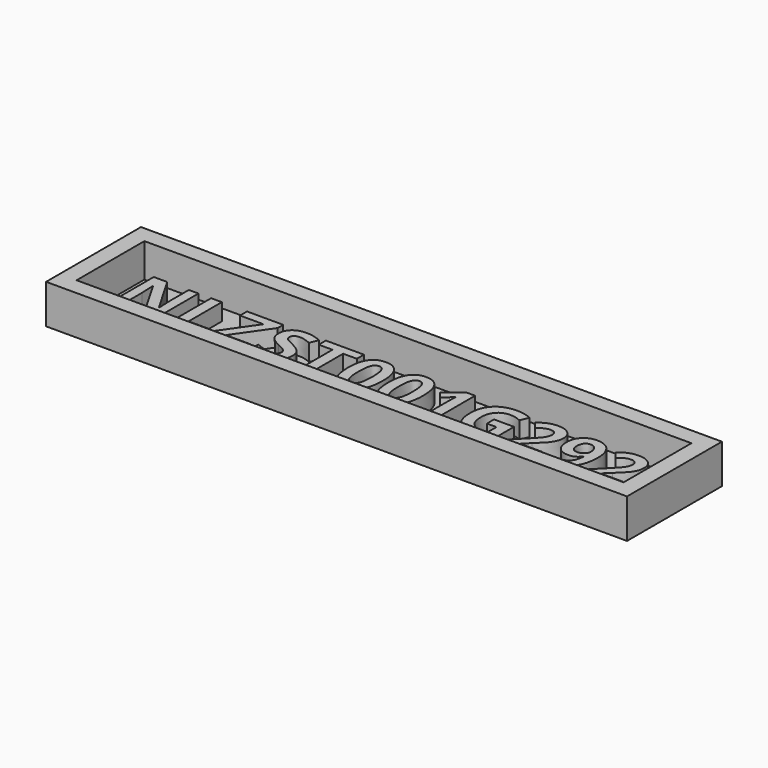
from build123d import *

# Parameters (mm, degrees)
F1_W          = 102.5095052083
F1_H          = 15.875
F2_DEPTH      = 1
F0_TEXT_SIZE  = 13.2291666667
F3_DEPTH      = 3.175
F4_W          = 108.8595052083
F4_H          = 22.225
F4_W_2        = 102.5095052083
F4_H_2        = 15.875
F5_DEPTH      = 6.35
F5_DEPTH_BACK = 1


# Not quite as in the source:
# - Text() gives the source's letters only with a copy of the font that has no kerning and outlines rounded to 1/6400 em; it was checked with that copy


with BuildPart() as f2:
    # F1 (on Top) → F2 (new body)
    with BuildSketch(Plane.XY):
        with Locations((-1.1097179826, 6.1376898289)):
            Rectangle(F1_W, F1_H)
    extrude(amount=-F2_DEPTH)

    # F0 (on Top) → F3 (join)
    with BuildSketch(Plane.XY):
        with Locations((-49.1894705868, 1.3751898289)):
            Text('NLZST001G292', F0_TEXT_SIZE, font='Open Sans', font_style=FontStyle.BOLD, text_align=(TextAlign.LEFT, TextAlign.BOTTOM))
    extrude(amount=F3_DEPTH)

    # F4 (on Top) → F5 (join, two sides)
    with BuildSketch(Plane.XY) as f5_sk:
        with Locations((-1.1097179826, 6.1376898289)):
            Rectangle(F4_W, F4_H)
        with Locations((-1.1097179826, 6.1376898289)):
            Rectangle(F4_W_2, F4_H_2, mode=Mode.SUBTRACT)
    extrude(amount=F5_DEPTH)
    extrude(f5_sk.sketch, amount=-F5_DEPTH_BACK)


solid = f2.part
